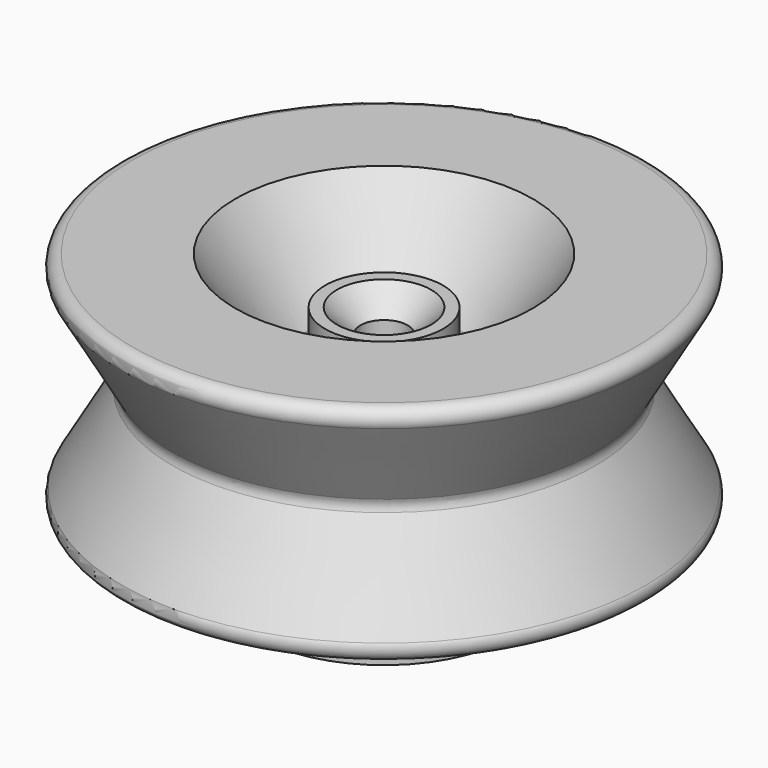
from build123d import *

# Parameters (mm, degrees)
F0_R     = 11
F0_R_2   = 6
F1_DEPTH = 6.95
F0_R_3   = 5
F0_R_4   = 3.8
F0_R_5   = 2
F2_DEPTH = 3
F5_START = -3
F5_DEPTH = 3
F6_R     = 1
F6_2_R   = 1
F7_START = 6.95
F7_DEPTH = 8.05
F8_DEPTH = 6.95
F9_SIZE  = 2
F12_R    = 5


# Not quite as in the source:
# - a fillet or chamfer that OpenCascade refuses, or shapes differently, is made with other operations: its cross-section is extruded or revolved along the edge and cut away or added
# - a feature of the source that left no trace in its solid (it failed there, or was rolled back) is left out


with BuildPart() as f1:
    # F0 (on Top) → F1 (new body)
    with BuildSketch(Plane.XY):
        Circle(F0_R)
        Circle(F0_R_2, mode=Mode.SUBTRACT)
    extrude(amount=F1_DEPTH)


with BuildPart() as f2:
    # F0 (on Top) → F2 (new body)
    with BuildSketch(Plane.XY):
        Circle(F0_R_2)
        Circle(F0_R_3, mode=Mode.SUBTRACT)
        Circle(F0_R_3)
        Circle(F0_R_4, mode=Mode.SUBTRACT)
        Circle(F0_R_4)
        Circle(F0_R_5, mode=Mode.SUBTRACT)
    extrude(amount=-F2_DEPTH)

    # F0 (on Top) → F5 (join)
    with BuildSketch(Plane.XY.offset(F5_START)):
        Circle(F0_R)
        Circle(F0_R_2, mode=Mode.SUBTRACT)
        Circle(F0_R_2)
        Circle(F0_R_3, mode=Mode.SUBTRACT)
        Circle(F0_R_3)
        Circle(F0_R_4, mode=Mode.SUBTRACT)
    extrude(amount=-F5_DEPTH)

    # F6
    f6_edges = [f2.edges().sort_by_distance(p)[0] for p in [
        (-11, 0, -3),
    ]]
    fillet(f6_edges, radius=F6_R)

    # F0 (on Top) → F8 (join, through all)
    with BuildSketch(Plane.XY):
        Circle(F0_R_4)
        Circle(F0_R_5, mode=Mode.SUBTRACT)
    extrude(amount=F8_DEPTH)

    # F10: fillet of radius 2 on 1 edges, made by hand

    # F10_s1 → F10_t2 (revolve)
    with BuildSketch(Plane.XZ):
        with BuildLine():
            ThreePointArc((2, -3), (3.2832396974, -3.6483340877), (3.8, -4.9899748742))
            Line((3.8, -4.9899748742), (3.8, -3))
            Line((3.8, -3), (2, -3))
        make_face()
    revolve(axis=Axis((0, 0, -3), (0, 0, 1)))


with BuildPart() as f4:
    # F3 (on Front) → F4 (revolve)
    with BuildSketch(Plane.XZ):
        Polygon((-17.6626499742, 9.5), (-23.107943549, 0), (-11.1, 0), (-11.1, 6.95), (-6, 6.95), (-6, 9.5009684645), (-12.6025350764, 19), (-23.107943549, 19), align=None)
    revolve(axis=Axis((0, 0, 9.5), (0, 0, -1)))

    # F6#2
    f6_2_edges = [f4.edges().sort_by_distance(p)[0] for p in [
        (23.107944, 0, 19),
        (23.107944, 0, 0),
        (17.66265, 0, 9.5),
    ]]
    fillet(f6_2_edges, radius=F6_2_R)

    # F12
    f12_edges = [f4.edges().sort_by_distance(p)[0] for p in [
        (6, 0, 9.500968),
    ]]
    fillet(f12_edges, radius=F12_R)


with BuildPart() as f7:
    # F0 (on Top) → F7 (new body)
    with BuildSketch(Plane.XY.offset(F7_START)):
        Circle(F0_R_3)
        Circle(F0_R_4, mode=Mode.SUBTRACT)
        Circle(F0_R_4)
        Circle(F0_R_5, mode=Mode.SUBTRACT)
    extrude(amount=F7_DEPTH)

    # F9
    f9_edges = [f7.edges().sort_by_distance(p)[0] for p in [
        (-2, 0, 15),
    ]]
    chamfer(f9_edges, length=F9_SIZE)


solid = Compound([f1.part, f2.part, f4.part, f7.part])
